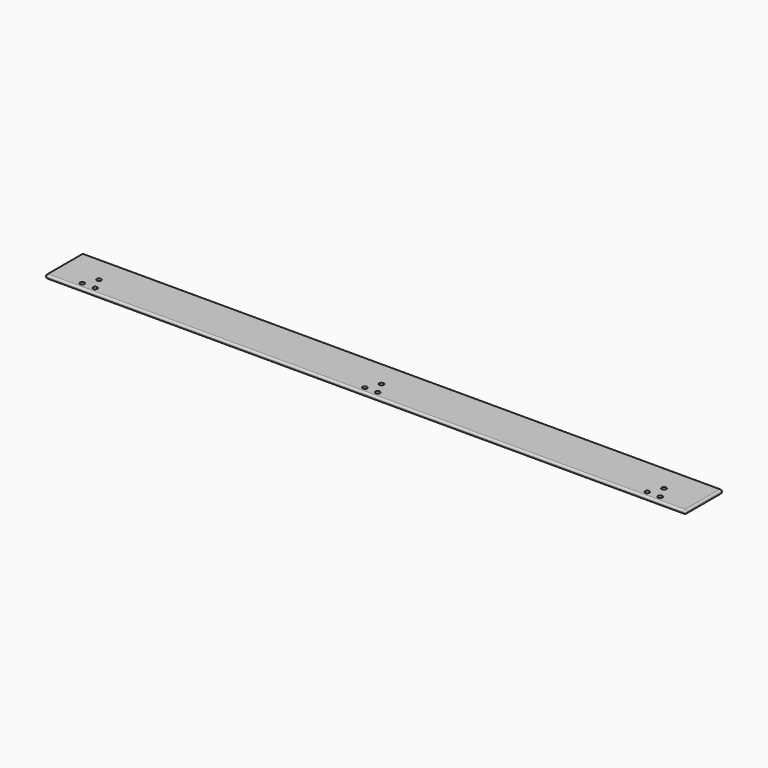
from build123d import *

# Parameters (mm, degrees)
F0_R     = 3.5
F1_DEPTH = 6
F2_R     = 2.99999


# Not quite as in the source:
# - a fillet or chamfer is up to 0.001 mm smaller than in the source, because OpenCascade refuses the exact size


with BuildPart() as f1:
    # F0 (on Top) → F1 (new body)
    with BuildSketch(Plane.XY):
        with BuildLine():
            Line((833.1764324449, 34.7622951977), (-158.1848585529, 34.7622951977))
            ThreePointArc((-158.1848585529, 34.7622951977), (-160.3061788964, 33.8836155413), (-161.1848585529, 31.7622951977))
            Line((-161.1848585529, 31.7622951977), (-161.1848585529, -35.2377048023))
            ThreePointArc((-161.1848585529, -35.2377048023), (-160.3061788964, -37.3590251459), (-158.1848585529, -38.2377048023))
            Line((-158.1848585529, -38.2377048023), (833.1764324449, -38.2377048023))
            ThreePointArc((833.1764324449, -38.2377048023), (835.2977527885, -37.3590251459), (836.1764324449, -35.2377048023))
            Line((836.1764324449, -35.2377048023), (836.1764324449, 31.7622951977))
            ThreePointArc((836.1764324449, 31.7622951977), (835.2977527885, 33.8836155413), (833.1764324449, 34.7622951977))
        make_face()
        with Locations((-111.1848585529, -28.2377048023)):
            Circle(F0_R, mode=Mode.SUBTRACT)
        with Locations((-91.1848585529, -28.2377048023)):
            Circle(F0_R, mode=Mode.SUBTRACT)
        with Locations((328.8151414471, -28.2377048023)):
            Circle(F0_R, mode=Mode.SUBTRACT)
        with Locations((-101.1848585529, -8.2377048023)):
            Circle(F0_R, mode=Mode.SUBTRACT)
        with Locations((348.8151414471, -28.2377048023)):
            Circle(F0_R, mode=Mode.SUBTRACT)
        with Locations((768.8151414471, -28.2377048023)):
            Circle(F0_R, mode=Mode.SUBTRACT)
        with Locations((788.8151414471, -28.2377048023)):
            Circle(F0_R, mode=Mode.SUBTRACT)
        with Locations((338.8151414471, -8.2377048023)):
            Circle(F0_R, mode=Mode.SUBTRACT)
        with Locations((778.8151414471, -8.2377048023)):
            Circle(F0_R, mode=Mode.SUBTRACT)
    extrude(amount=F1_DEPTH)

    # F2 (radius 3 in the source; OpenCascade refuses exactly that, so slightly less here)
    f2_edges = [f1.edges().sort_by_distance(p)[0] for p in [
        (836.176432, -35.237705, 3),
        (836.176432, 31.762295, 3),
        (836.176432, -1.737705, 0),
        (836.176432, -1.737705, 6),
    ]]
    fillet(f2_edges, radius=F2_R)


solid = f1.part
